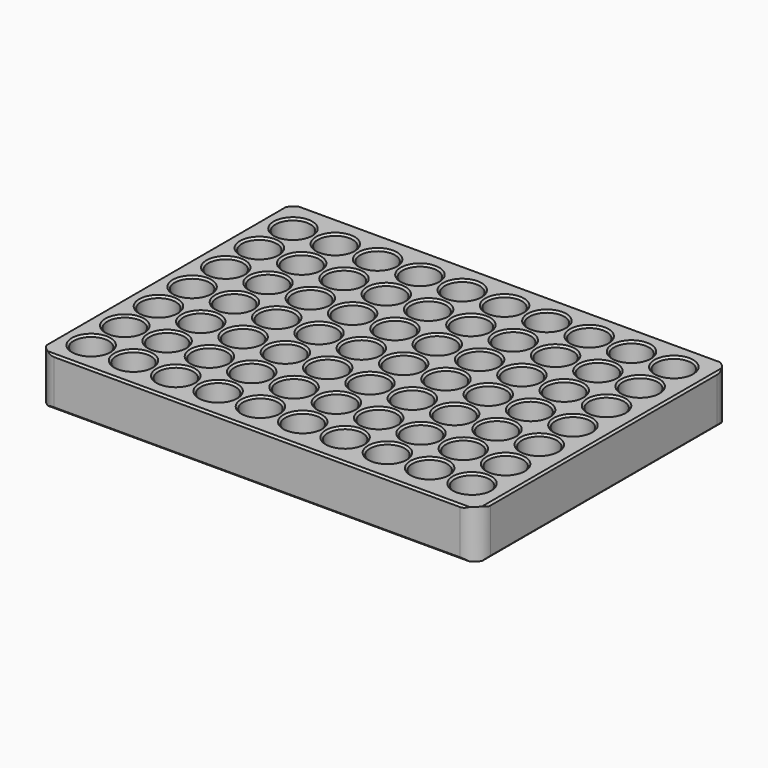
from build123d import *

# Parameters (mm, degrees)
F0_W        = 183
F0_H        = 132
F0_R        = 7.25
F1_DEPTH    = 20
F2_SIZE     = 0.8
F3_T1_DEPTH = 53.4


# Not quite as in the source:
# - a fillet or chamfer that OpenCascade refuses, or shapes differently, is made with other operations: its cross-section is extruded or revolved along the edge and cut away or added


with BuildPart() as f1:
    # F0 (on Top) → F1 (new body)
    with BuildSketch(Plane.XY):
        with Locations((13.4596604586, 66)):
            Rectangle(F0_W, F0_H)
        with Locations((-65.9653395414, 12.925)):
            Circle(F0_R, mode=Mode.SUBTRACT)
        with Locations((-48.4659155486, 13.0669856336)):
            Circle(F0_R, mode=Mode.SUBTRACT)
        with Locations((-65.9653395414, 30.425)):
            Circle(F0_R, mode=Mode.SUBTRACT)
        with Locations((-48.4659155486, 30.5669856336)):
            Circle(F0_R, mode=Mode.SUBTRACT)
        with Locations((-30.9664915558, 13.2089712672)):
            Circle(F0_R, mode=Mode.SUBTRACT)
        with Locations((-13.467067563, 13.3509569008)):
            Circle(F0_R, mode=Mode.SUBTRACT)
        with Locations((4.0323564298, 13.4929425344)):
            Circle(F0_R, mode=Mode.SUBTRACT)
        with Locations((-30.9664915558, 30.7089712672)):
            Circle(F0_R, mode=Mode.SUBTRACT)
        with Locations((-13.467067563, 30.8509569008)):
            Circle(F0_R, mode=Mode.SUBTRACT)
        with Locations((4.0323564298, 30.9929425344)):
            Circle(F0_R, mode=Mode.SUBTRACT)
        with Locations((-65.9653395414, 47.925)):
            Circle(F0_R, mode=Mode.SUBTRACT)
        with Locations((-48.4659155486, 48.0669856336)):
            Circle(F0_R, mode=Mode.SUBTRACT)
        with Locations((-65.9653395414, 65.425)):
            Circle(F0_R, mode=Mode.SUBTRACT)
        with Locations((-48.4659155486, 65.5669856336)):
            Circle(F0_R, mode=Mode.SUBTRACT)
        with Locations((-30.9664915558, 48.2089712672)):
            Circle(F0_R, mode=Mode.SUBTRACT)
        with Locations((-13.467067563, 48.3509569008)):
            Circle(F0_R, mode=Mode.SUBTRACT)
        with Locations((4.0323564298, 48.4929425344)):
            Circle(F0_R, mode=Mode.SUBTRACT)
        with Locations((-30.9664915558, 65.7089712672)):
            Circle(F0_R, mode=Mode.SUBTRACT)
        with Locations((-13.467067563, 65.8509569008)):
            Circle(F0_R, mode=Mode.SUBTRACT)
        with Locations((4.0323564298, 65.9929425344)):
            Circle(F0_R, mode=Mode.SUBTRACT)
        with Locations((21.5317804226, 13.634928168)):
            Circle(F0_R, mode=Mode.SUBTRACT)
        with Locations((39.0312044154, 13.7769138016)):
            Circle(F0_R, mode=Mode.SUBTRACT)
        with Locations((56.5306284082, 13.9188994352)):
            Circle(F0_R, mode=Mode.SUBTRACT)
        with Locations((21.5317804226, 31.134928168)):
            Circle(F0_R, mode=Mode.SUBTRACT)
        with Locations((39.0312044154, 31.2769138016)):
            Circle(F0_R, mode=Mode.SUBTRACT)
        with Locations((56.5306284082, 31.4188994352)):
            Circle(F0_R, mode=Mode.SUBTRACT)
        with Locations((74.030052401, 14.0608850688)):
            Circle(F0_R, mode=Mode.SUBTRACT)
        with Locations((91.5294763938, 14.2028707024)):
            Circle(F0_R, mode=Mode.SUBTRACT)
        with Locations((74.030052401, 31.5608850688)):
            Circle(F0_R, mode=Mode.SUBTRACT)
        with Locations((91.5294763938, 31.7028707024)):
            Circle(F0_R, mode=Mode.SUBTRACT)
        with Locations((21.5317804226, 48.634928168)):
            Circle(F0_R, mode=Mode.SUBTRACT)
        with Locations((39.0312044154, 48.7769138016)):
            Circle(F0_R, mode=Mode.SUBTRACT)
        with Locations((56.5306284082, 48.9188994352)):
            Circle(F0_R, mode=Mode.SUBTRACT)
        with Locations((74.030052401, 49.0608850688)):
            Circle(F0_R, mode=Mode.SUBTRACT)
        with Locations((91.5294763938, 49.2028707024)):
            Circle(F0_R, mode=Mode.SUBTRACT)
        with Locations((-65.9653395414, 82.925)):
            Circle(F0_R, mode=Mode.SUBTRACT)
        with Locations((-48.4659155486, 83.0669856336)):
            Circle(F0_R, mode=Mode.SUBTRACT)
        with Locations((-30.9664915558, 83.2089712672)):
            Circle(F0_R, mode=Mode.SUBTRACT)
        with Locations((-13.467067563, 83.3509569008)):
            Circle(F0_R, mode=Mode.SUBTRACT)
        with Locations((4.0323564298, 83.4929425344)):
            Circle(F0_R, mode=Mode.SUBTRACT)
        with Locations((-65.9653395414, 100.425)):
            Circle(F0_R, mode=Mode.SUBTRACT)
        with Locations((-48.4659155486, 100.5669856336)):
            Circle(F0_R, mode=Mode.SUBTRACT)
        with Locations((-65.9653395414, 117.925)):
            Circle(F0_R, mode=Mode.SUBTRACT)
        with Locations((-48.4659155486, 118.0669856336)):
            Circle(F0_R, mode=Mode.SUBTRACT)
        with Locations((-30.9664915558, 100.7089712672)):
            Circle(F0_R, mode=Mode.SUBTRACT)
        with Locations((-13.467067563, 100.8509569008)):
            Circle(F0_R, mode=Mode.SUBTRACT)
        with Locations((4.0323564298, 100.9929425344)):
            Circle(F0_R, mode=Mode.SUBTRACT)
        with Locations((-30.9664915558, 118.2089712672)):
            Circle(F0_R, mode=Mode.SUBTRACT)
        with Locations((-13.467067563, 118.3509569008)):
            Circle(F0_R, mode=Mode.SUBTRACT)
        with Locations((4.0323564298, 118.4929425344)):
            Circle(F0_R, mode=Mode.SUBTRACT)
        with Locations((21.5317804226, 66.134928168)):
            Circle(F0_R, mode=Mode.SUBTRACT)
        with Locations((39.0312044154, 66.2769138016)):
            Circle(F0_R, mode=Mode.SUBTRACT)
        with Locations((56.5306284082, 66.4188994352)):
            Circle(F0_R, mode=Mode.SUBTRACT)
        with Locations((21.5317804226, 83.634928168)):
            Circle(F0_R, mode=Mode.SUBTRACT)
        with Locations((39.0312044154, 83.7769138016)):
            Circle(F0_R, mode=Mode.SUBTRACT)
        with Locations((56.5306284082, 83.9188994352)):
            Circle(F0_R, mode=Mode.SUBTRACT)
        with Locations((74.030052401, 66.5608850688)):
            Circle(F0_R, mode=Mode.SUBTRACT)
        with Locations((91.5294763938, 66.7028707024)):
            Circle(F0_R, mode=Mode.SUBTRACT)
        with Locations((74.030052401, 84.0608850688)):
            Circle(F0_R, mode=Mode.SUBTRACT)
        with Locations((91.5294763938, 84.2028707024)):
            Circle(F0_R, mode=Mode.SUBTRACT)
        with Locations((21.5317804226, 101.134928168)):
            Circle(F0_R, mode=Mode.SUBTRACT)
        with Locations((39.0312044154, 101.2769138016)):
            Circle(F0_R, mode=Mode.SUBTRACT)
        with Locations((56.5306284082, 101.4188994352)):
            Circle(F0_R, mode=Mode.SUBTRACT)
        with Locations((21.5317804226, 118.634928168)):
            Circle(F0_R, mode=Mode.SUBTRACT)
        with Locations((39.0312044154, 118.7769138016)):
            Circle(F0_R, mode=Mode.SUBTRACT)
        with Locations((56.5306284082, 118.9188994352)):
            Circle(F0_R, mode=Mode.SUBTRACT)
        with Locations((74.030052401, 101.5608850688)):
            Circle(F0_R, mode=Mode.SUBTRACT)
        with Locations((91.5294763938, 101.7028707024)):
            Circle(F0_R, mode=Mode.SUBTRACT)
        with Locations((74.030052401, 119.0608850688)):
            Circle(F0_R, mode=Mode.SUBTRACT)
        with Locations((91.5294763938, 119.2028707024)):
            Circle(F0_R, mode=Mode.SUBTRACT)
    extrude(amount=F1_DEPTH)

    # F2
    f2_edges = [f1.edges().sort_by_distance(p)[0] for p in [
        (13.45966, 0, 20),
        (104.95966, 66, 20),
        (13.45966, 132, 20),
        (-78.04034, 66, 20),
        (-73.21534, 12.925, 20),
        (-55.715916, 13.066986, 20),
        (-73.21534, 30.425, 20),
        (-55.715916, 30.566986, 20),
        (-38.216492, 13.208971, 20),
        (-20.717068, 13.350957, 20),
        (-3.217644, 13.492943, 20),
        (-38.216492, 30.708971, 20),
        (-20.717068, 30.850957, 20),
        (-3.217644, 30.992943, 20),
        (-73.21534, 47.925, 20),
        (-55.715916, 48.066986, 20),
        (-73.21534, 65.425, 20),
        (-55.715916, 65.566986, 20),
        (-38.216492, 48.208971, 20),
        (-20.717068, 48.350957, 20),
        (-3.217644, 48.492943, 20),
        (-38.216492, 65.708971, 20),
        (-20.717068, 65.850957, 20),
        (-3.217644, 65.992943, 20),
        (14.28178, 13.634928, 20),
        (31.781204, 13.776914, 20),
        (49.280628, 13.918899, 20),
        (14.28178, 31.134928, 20),
        (31.781204, 31.276914, 20),
        (49.280628, 31.418899, 20),
        (66.780052, 14.060885, 20),
        (84.279476, 14.202871, 20),
        (66.780052, 31.560885, 20),
        (84.279476, 31.702871, 20),
        (14.28178, 48.634928, 20),
        (31.781204, 48.776914, 20),
        (49.280628, 48.918899, 20),
        (66.780052, 49.060885, 20),
        (84.279476, 49.202871, 20),
        (-73.21534, 82.925, 20),
        (-55.715916, 83.066986, 20),
        (-38.216492, 83.208971, 20),
        (-20.717068, 83.350957, 20),
        (-3.217644, 83.492943, 20),
        (-73.21534, 100.425, 20),
        (-55.715916, 100.566986, 20),
        (-73.21534, 117.925, 20),
        (-55.715916, 118.066986, 20),
        (-38.216492, 100.708971, 20),
        (-20.717068, 100.850957, 20),
        (-3.217644, 100.992943, 20),
        (-38.216492, 118.208971, 20),
        (-20.717068, 118.350957, 20),
        (-3.217644, 118.492943, 20),
        (14.28178, 66.134928, 20),
        (31.781204, 66.276914, 20),
        (49.280628, 66.418899, 20),
        (14.28178, 83.634928, 20),
        (31.781204, 83.776914, 20),
        (49.280628, 83.918899, 20),
        (66.780052, 66.560885, 20),
        (84.279476, 66.702871, 20),
        (66.780052, 84.060885, 20),
        (84.279476, 84.202871, 20),
        (14.28178, 101.134928, 20),
        (31.781204, 101.276914, 20),
        (49.280628, 101.418899, 20),
        (14.28178, 118.634928, 20),
        (31.781204, 118.776914, 20),
        (49.280628, 118.918899, 20),
        (66.780052, 101.560885, 20),
        (84.279476, 101.702871, 20),
        (66.780052, 119.060885, 20),
        (84.279476, 119.202871, 20),
        (13.45966, 0, 0),
        (104.95966, 66, 0),
        (13.45966, 132, 0),
        (-78.04034, 66, 0),
        (-73.21534, 12.925, 0),
        (-55.715916, 13.066986, 0),
        (-73.21534, 30.425, 0),
        (-55.715916, 30.566986, 0),
        (-38.216492, 13.208971, 0),
        (-20.717068, 13.350957, 0),
        (-3.217644, 13.492943, 0),
        (-38.216492, 30.708971, 0),
        (-20.717068, 30.850957, 0),
        (-3.217644, 30.992943, 0),
        (-73.21534, 47.925, 0),
        (-55.715916, 48.066986, 0),
        (-73.21534, 65.425, 0),
        (-55.715916, 65.566986, 0),
        (-38.216492, 48.208971, 0),
        (-20.717068, 48.350957, 0),
        (-3.217644, 48.492943, 0),
        (-38.216492, 65.708971, 0),
        (-20.717068, 65.850957, 0),
        (-3.217644, 65.992943, 0),
        (14.28178, 13.634928, 0),
        (31.781204, 13.776914, 0),
        (49.280628, 13.918899, 0),
        (14.28178, 31.134928, 0),
        (31.781204, 31.276914, 0),
        (49.280628, 31.418899, 0),
        (66.780052, 14.060885, 0),
        (84.279476, 14.202871, 0),
        (66.780052, 31.560885, 0),
        (84.279476, 31.702871, 0),
        (14.28178, 48.634928, 0),
        (31.781204, 48.776914, 0),
        (49.280628, 48.918899, 0),
        (66.780052, 49.060885, 0),
        (84.279476, 49.202871, 0),
        (-73.21534, 82.925, 0),
        (-55.715916, 83.066986, 0),
        (-38.216492, 83.208971, 0),
        (-20.717068, 83.350957, 0),
        (-3.217644, 83.492943, 0),
        (-73.21534, 100.425, 0),
        (-55.715916, 100.566986, 0),
        (-73.21534, 117.925, 0),
        (-55.715916, 118.066986, 0),
        (-38.216492, 100.708971, 0),
        (-20.717068, 100.850957, 0),
        (-3.217644, 100.992943, 0),
        (-38.216492, 118.208971, 0),
        (-20.717068, 118.350957, 0),
        (-3.217644, 118.492943, 0),
        (14.28178, 66.134928, 0),
        (31.781204, 66.276914, 0),
        (49.280628, 66.418899, 0),
        (14.28178, 83.634928, 0),
        (31.781204, 83.776914, 0),
        (49.280628, 83.918899, 0),
        (66.780052, 66.560885, 0),
        (84.279476, 66.702871, 0),
        (66.780052, 84.060885, 0),
        (84.279476, 84.202871, 0),
        (14.28178, 101.134928, 0),
        (31.781204, 101.276914, 0),
        (49.280628, 101.418899, 0),
        (14.28178, 118.634928, 0),
        (31.781204, 118.776914, 0),
        (49.280628, 118.918899, 0),
        (66.780052, 101.560885, 0),
        (84.279476, 101.702871, 0),
        (66.780052, 119.060885, 0),
        (84.279476, 119.202871, 0),
    ]]
    chamfer(f2_edges, length=F2_SIZE)

    # F3: fillet of radius 7 on 4 edges, made by hand

    # F3_s2 → F3_t1 (cut)
    with BuildSketch(Plane.XY.offset(-16.7)):
        with BuildLine():
            ThreePointArc((-71.0403395414, 0), (-75.9900870097, 2.0502525317), (-78.0403395414, 7))
            Line((-78.0403395414, 7), (-78.0403395414, 0))
            Line((-78.0403395414, 0), (-71.0403395414, 0))
        make_face()
        with BuildLine():
            ThreePointArc((97.9596604586, 0), (102.9094079269, 2.0502525317), (104.9596604586, 7))
            Line((104.9596604586, 7), (104.9596604586, 0))
            Line((104.9596604586, 0), (97.9596604586, 0))
        make_face()
        with BuildLine():
            ThreePointArc((104.9596604586, 125), (102.9094079269, 129.9497474683), (97.9596604586, 132))
            Line((97.9596604586, 132), (104.9596604586, 132))
            Line((104.9596604586, 132), (104.9596604586, 125))
        make_face()
        with BuildLine():
            ThreePointArc((-78.0403395414, 125), (-75.9900870097, 129.9497474683), (-71.0403395414, 132))
            Line((-71.0403395414, 132), (-78.0403395414, 132))
            Line((-78.0403395414, 132), (-78.0403395414, 125))
        make_face()
    extrude(amount=F3_T1_DEPTH, mode=Mode.SUBTRACT)


solid = f1.part
